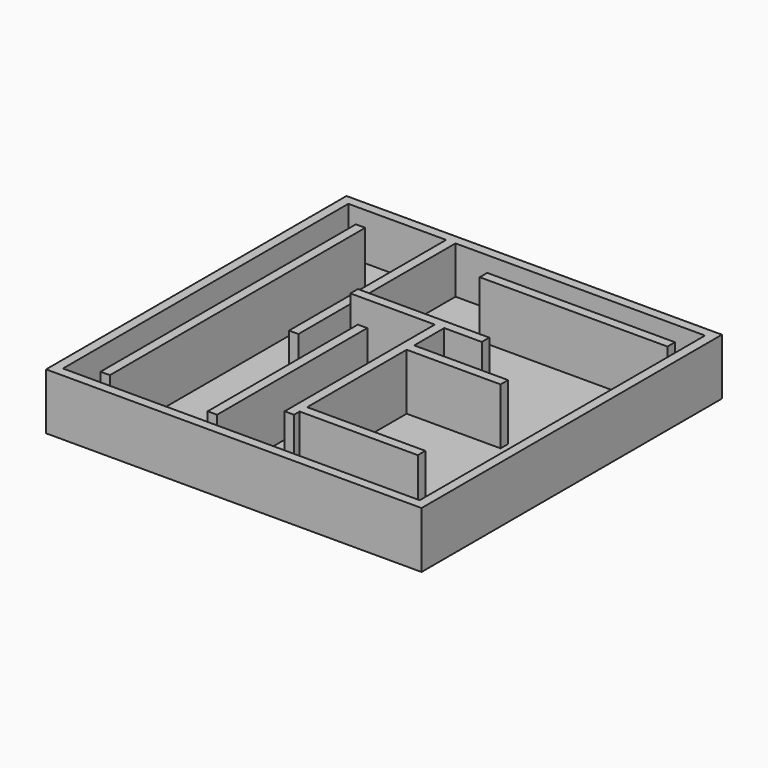
from build123d import *

# Parameters (mm, degrees)
F0_W      = 50.8
F0_H      = 50.8
F1_DEPTH  = 7.62
F2_T      = -1.27
F3_W      = 1.27
F3_H      = 43.18
F4_DEPTH  = 7.62
F5_W      = 1.27
F5_H      = 26.6756825149
F6_DEPTH  = 7.62
F7_W      = 1.27
F7_H      = 25.4
F8_DEPTH  = 7.62
F9_W      = 17.78
F9_H      = 1.27
F10_DEPTH = 7.62
F11_W     = 1.27
F11_H     = 25.4
F12_DEPTH = 7.62
F13_W     = 12.7
F13_H     = 1.27
F14_DEPTH = 7.62
F15_W     = 15.9816620052
F15_H     = 1.27
F16_DEPTH = 7.62
F17_W     = 25.4
F17_H     = 1.27
F18_DEPTH = 7.62
F19_R     = 1.27
F20_DEPTH = 203.2


# Not quite as in the source:
# - a feature names something its author has since deleted; it is built from what else it names


with BuildPart() as f1:
    # F0 (on Top) → F1 (new body)
    with BuildSketch(Plane.XY):
        with Locations((25.4, 25.4)):
            Rectangle(F0_W, F0_H)
    extrude(amount=-F1_DEPTH)

    # F2
    f2_openings = [f1.faces().sort_by_distance(p)[0] for p in [
        (25.4, 25.4, 0),
    ]]
    offset(amount=F2_T, openings=f2_openings)

    # F3 (on face) → F4 (join)
    with BuildSketch(Plane.XY.offset(-6.35)):
        with Locations((6.985, 22.86)):
            Rectangle(F3_W, F3_H)
    extrude(amount=F4_DEPTH)

    # F5 (on Top) → F6 (join)
    with BuildSketch(Plane.XY):
        with Locations((15.1333379948, 36.3023299724)):
            Rectangle(F5_W, F5_H)
    extrude(amount=-F6_DEPTH)

    # F7 (on face) → F8 (join)
    with BuildSketch(Plane.XY.offset(-6.35)):
        with Locations((21.4833379948, 13.97)):
            Rectangle(F7_W, F7_H)
    extrude(amount=F8_DEPTH)

    # F9 (on face) → F10 (join)
    with BuildSketch(Plane.XY.offset(-6.35)):
        with Locations((24.6583379948, 32.385)):
            Rectangle(F9_W, F9_H)
    extrude(amount=F10_DEPTH)

    # F11 (on face) → F12 (join)
    with BuildSketch(Plane.XY.offset(-6.35)):
        with Locations((27.8333379948, 19.05)):
            Rectangle(F11_W, F11_H)
    extrude(amount=F12_DEPTH)

    # F13 (on face) → F14 (join)
    with BuildSketch(Plane.XY.offset(-6.35)):
        with Locations((34.8183379948, 26.035)):
            Rectangle(F13_W, F13_H)
    extrude(amount=F14_DEPTH)

    # F15 (on face) → F16 (join)
    with BuildSketch(Plane.XY.offset(-6.35)):
        with Locations((36.4591689974, 7.9343094056)):
            Rectangle(F15_W, F15_H)
    extrude(amount=F16_DEPTH)

    # F17 (on face) → F18 (join)
    with BuildSketch(Plane.XY.offset(-6.35)):
        with Locations((36.83, 43.815)):
            Rectangle(F17_W, F17_H)
    extrude(amount=F18_DEPTH)

    # F19 (on face) → F20 (cut)
    with BuildSketch(Plane.XY.offset(-6.35)):
        with Locations((3.6000448745, 4.547465127)):
            Circle(F19_R)
        with Locations((3.8395691663, 10.7227088884)):
            Circle(F19_R)
        with Locations((19.5783379948, 36.2029448152)):
            Circle(F19_R)
        with Locations((31.4771048725, 16.6409648955)):
            Circle(F19_R)
    extrude(amount=-F20_DEPTH, mode=Mode.SUBTRACT)


solid = f1.part
